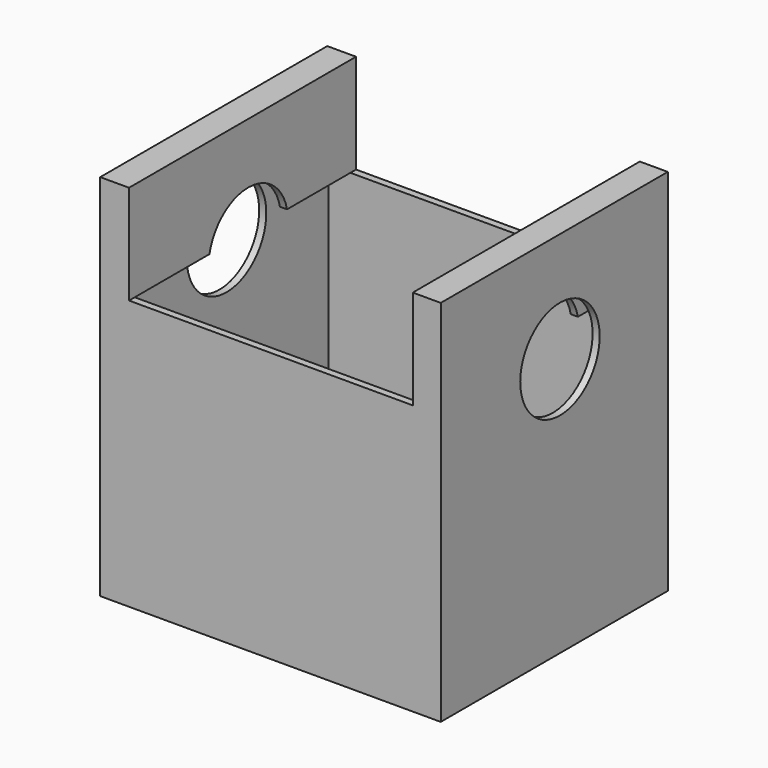
from build123d import *

# Parameters (mm, degrees)
F0_W     = 120
F0_H     = 130
F1_DEPTH = 100
F2_W     = 100
F2_H     = 35
F3_DEPTH = 125
F4_T     = -2.5
F5_R     = 17.5
F6_DEPTH = 5005


# Not quite as in the source:
# - a shell that OpenCascade refuses in one call is made with other operations: the cavity is built on its own and cut out


with BuildPart() as f1:
    # F0 (on Front) → F1 (new body)
    with BuildSketch(Plane.XZ):
        with Locations((-0.7081851363, 2.2362722828)):
            Rectangle(F0_W, F0_H)
    extrude(amount=F1_DEPTH)

    # F2 (on face) → F3 (cut)
    with BuildSketch(Plane.XZ.offset(100)):
        with Locations((-0.5643002689, 49.7362722828)):
            Rectangle(F2_W, F2_H)
    extrude(amount=-F3_DEPTH, mode=Mode.SUBTRACT)

    # F4: a shell. OpenCascade refuses it in one call, so the cavity is built on its own and cut out:
    # the body offset inwards by the wall thickness, plus a prism from it out through each open face.
    f4_core = offset(f1.part, amount=F4_T, kind=Kind.INTERSECTION, mode=Mode.PRIVATE)
    f4_exits = [f4_core.faces().sort_by_distance(p)[0] for p in [
        (-0.5643, -50, 29.736272),
    ]]
    add(f4_core, mode=Mode.SUBTRACT)
    extrude(f4_exits, amount=-F4_T, mode=Mode.SUBTRACT)

    # F5 (on face) → F6 (cut)
    with BuildSketch(Plane(origin=(-60.7081851363, 0, 0), x_dir=(0, -1, 0), z_dir=(-1, 0, 0))):
        with Locations((47.4842637777, 28.4689757973)):
            Circle(F5_R)
    extrude(amount=-F6_DEPTH, mode=Mode.SUBTRACT)


solid = f1.part
